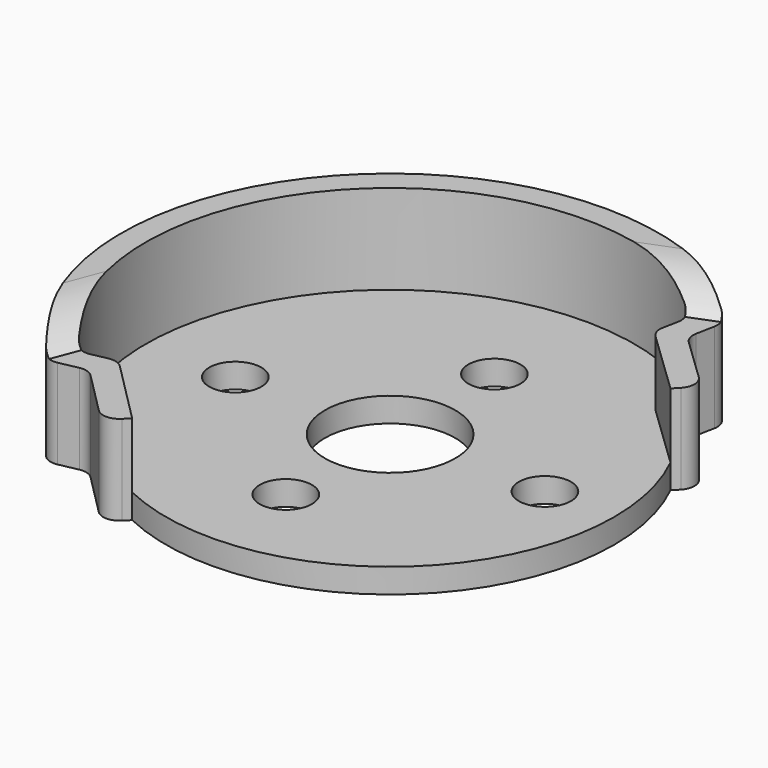
from build123d import *

# Parameters (mm, degrees)
F1_DEPTH    = 1.5
F2_DEPTH    = 5.5
F3_DEPTH    = 7
F4_T1_DEPTH = 21.6191756982
F4_T3_DEPTH = 21.6239840214
F5_R        = 1
F6_D        = 3.2
F6_DEPTH    = 4
F6_TIP      = 0.9613769904
F7_D        = 8
F7_DEPTH    = 4
F7_TIP      = 2.4034424761


# Not quite as in the source:
# - a fillet or chamfer that OpenCascade refuses, or shapes differently, is made with other operations: its cross-section is extruded or revolved along the edge and cut away or added


with BuildPart() as f1:
    # F0 (on Top) → F1 (new body)
    with BuildSketch(Plane.XY):
        with BuildLine():
            Line((-66.0687833834, 84.994474126), (-65.6429035596, 87.1528592574))
            ThreePointArc((-65.6429035596, 87.1528592574), (-84.7546054832, 85.2563072371), (-86.3354477268, 66.1159050004))
            Line((-86.3354477268, 66.1159050004), (-84.1804171789, 66.558446905))
            Line((-84.1804171789, 66.558446905), (-79.945453805, 62.3081427722))
            ThreePointArc((-79.945453805, 62.3081427722), (-64.2506598446, 65.1001279098), (-61.7378264361, 80.8420276277))
            Line((-61.7378264361, 80.8420276277), (-66.0687833834, 84.994474126))
        make_face()
    extrude(amount=F1_DEPTH)

    # F0 (on Top) → F2 (join)
    with BuildSketch(Plane.XY):
        Polygon((-84.1804171789, 66.558446905), (-86.3354477268, 66.1159050004), (-86.9652344199, 64.4552756389), (-84.6716307932, 64.9262739357), (-81.0080298382, 61.2494019287), (-79.945453805, 62.3081427722), align=None)
        Polygon((-63.9854566278, 87.8042374119), (-65.6429035596, 87.1528592574), (-66.0687833834, 84.994474126), (-61.7378264361, 80.8420276277), (-60.6997148116, 81.9247668645), (-64.4382903395, 85.5092483194), align=None)
    extrude(amount=F2_DEPTH)

    # F0 (on Top) → F3 (join)
    with BuildSketch(Plane.XY):
        with BuildLine():
            ThreePointArc((-86.3354477268, 66.1159050004), (-84.7546054832, 85.2563072371), (-65.6429035596, 87.1528592574))
            Line((-65.6429035596, 87.1528592574), (-63.9854566278, 87.8042374119))
            ThreePointArc((-63.9854566278, 87.8042374119), (-85.82068996, 86.3115247186), (-86.9652344199, 64.4552756389))
            Line((-86.9652344199, 64.4552756389), (-86.3354477268, 66.1159050004))
        make_face()
    extrude(amount=F3_DEPTH)

    # F4: fillet of radius 6 on 2 edges, made by hand

    # F4_s2 → F4_t1 (cut)
    with BuildSketch(Plane(origin=(6.9172981305, 18.2396174816, 0), x_dir=(0, 0, 1), z_dir=(0.3546014652, 0.9350175404, 0))):
        with BuildLine():
            ThreePointArc((5.5, -104.169954771), (6.6124860802, -106.0172613941), (7, -108.1385817376))
            Line((7, -108.1385817376), (7, -104.169954771))
            Line((7, -104.169954771), (5.5, -104.169954771))
        make_face()
    extrude(amount=F4_T1_DEPTH, mode=Mode.SUBTRACT)

    # F4_s4 → F4_t3 (cut)
    with BuildSketch(Plane(origin=(-36.4260217608, -14.315459745, 0), x_dir=(0, 0, 1), z_dir=(0.9307059478, 0.3657682856, 0))):
        with BuildLine():
            ThreePointArc((5.5, -105.123776774), (6.6124860802, -106.971083397), (7, -109.0924037406))
            Line((7, -109.0924037406), (7, -105.123776774))
            Line((7, -105.123776774), (5.5, -105.123776774))
        make_face()
    extrude(amount=F4_T3_DEPTH, mode=Mode.SUBTRACT)

    # F5 (call 1 of 10: OpenCascade refuses the feature's edges together)
    f5_edges = [f1.edges().sort_by_distance(p)[0] for p in [
        (-86.965234, 64.455276, 2.75),
    ]]
    fillet(f5_edges, radius=F5_R)

    # F5#2 (call 2 of 10)
    f5_2_edges = [f1.edges().sort_by_distance(p)[0] for p in [
        (-84.671631, 64.926274, 2.75),
    ]]
    fillet(f5_2_edges, radius=F5_R)

    # F5#3 (call 3 of 10)
    f5_3_edges = [f1.edges().sort_by_distance(p)[0] for p in [
        (-81.00803, 61.249402, 2.75),
    ]]
    fillet(f5_3_edges, radius=F5_R)

    # F5#4 (call 4 of 10)
    f5_4_edges = [f1.edges().sort_by_distance(p)[0] for p in [
        (-60.699715, 81.924767, 2.75),
    ]]
    fillet(f5_4_edges, radius=F5_R)

    # F5#5 (call 5 of 10)
    f5_5_edges = [f1.edges().sort_by_distance(p)[0] for p in [
        (-64.43829, 85.509248, 2.75),
    ]]
    fillet(f5_5_edges, radius=F5_R)

    # F5#6 (call 6 of 10)
    f5_6_edges = [f1.edges().sort_by_distance(p)[0] for p in [
        (-63.985457, 87.804237, 2.75),
    ]]
    fillet(f5_6_edges, radius=F5_R)

    # F5#7 (call 7 of 10)
    f5_7_edges = [f1.edges().sort_by_distance(p)[0] for p in [
        (-84.180417, 66.558447, 3.5),
    ]]
    fillet(f5_7_edges, radius=F5_R)

    # F5#8 (call 8 of 10)
    f5_8_edges = [f1.edges().sort_by_distance(p)[0] for p in [
        (-66.068783, 84.994474, 3.5),
    ]]
    fillet(f5_8_edges, radius=F5_R)

    # F5#9 (call 9 of 10)
    f5_9_edges = [f1.edges().sort_by_distance(p)[0] for p in [
        (-65.642904, 87.152859, 3.5),
    ]]
    fillet(f5_9_edges, radius=F5_R)

    # F5#10 (call 10 of 10)
    f5_10_edges = [f1.edges().sort_by_distance(p)[0] for p in [
        (-86.335448, 66.115905, 3.5),
    ]]
    fillet(f5_10_edges, radius=F5_R)

    # F6
    with Locations(Plane(origin=(0, 0, 0), x_dir=(1, 0, 0), z_dir=(0, 0, -1))):
        with Locations((-83.5608274937, -74.7376042604), (-74.0608274937, -82.7376042604), (-64.5608274937, -74.7376042604), (-74.0608274937, -66.7376042604)):
            Hole(F6_D / 2, depth=F6_DEPTH)
            with Locations((0, 0, -(F6_DEPTH + F6_TIP / 2))):  # 118° drill point
                Cone(0, F6_D / 2, F6_TIP, mode=Mode.SUBTRACT)

    # F7
    with Locations(Plane(origin=(0, 0, 0), x_dir=(1, 0, 0), z_dir=(0, 0, -1))):
        with Locations((-74.0608274937, -74.7376042604)):
            Hole(F7_D / 2, depth=F7_DEPTH)
            with Locations((0, 0, -(F7_DEPTH + F7_TIP / 2))):  # 118° drill point
                Cone(0, F7_D / 2, F7_TIP, mode=Mode.SUBTRACT)


solid = f1.part
